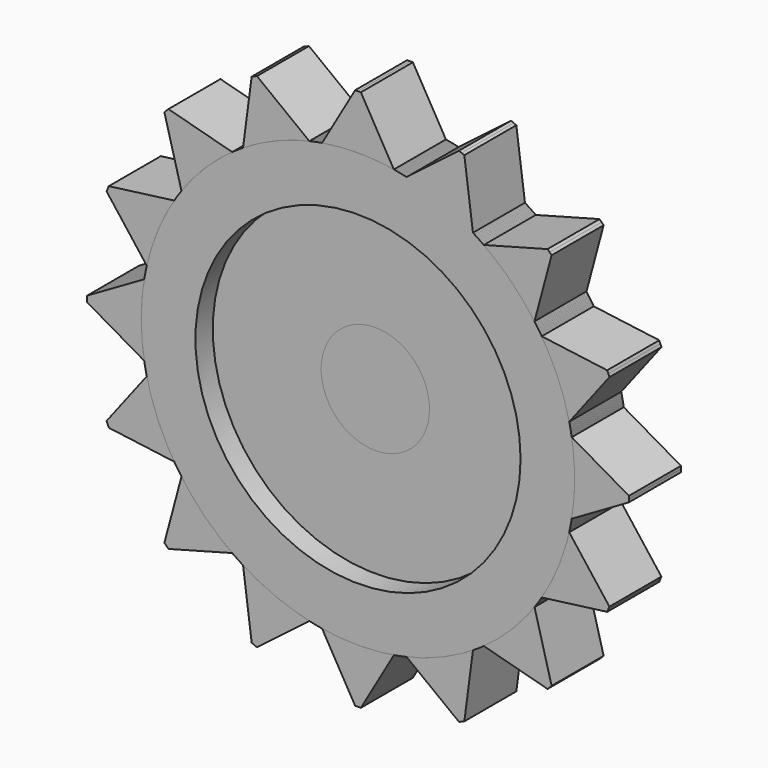
from build123d import *

# Parameters (mm, degrees)
F0_R     = 100
F1_DEPTH = 30
F3_DEPTH = 30
F5_COUNT = 16
F6_R     = 25
F7_DEPTH = 50
F8_R     = 75
F9_DEPTH = 10


# Not quite as in the source:
# - a feature of the source that left no trace in its solid (it failed there, or was rolled back) is left out


with BuildPart() as f1:
    # F0 (on Front) → F1 (new body)
    with BuildSketch(Plane.XZ):
        Circle(F0_R)
    extrude(amount=-F1_DEPTH)

    # F2 (on face) → F3 (join)
    with BuildSketch(Plane.XZ):
        Polygon((1.3260585624, 124.9999999801), (1.4569e-06, 125), (-1.32605566, 125), (-16.5566256365, 98.6198669008), (16.5566285461, 98.6198664123), align=None)
    extrude(amount=-F3_DEPTH)


with BuildPart() as f5_1:
    # F5: instance of F1
    add(f1.part.rotate(Axis((0, 2.4381279945, 0), (0, -1, 0)), 1 * 360 / F5_COUNT))


with BuildPart() as f5_2:
    # F5: instance of F1
    add(f1.part.rotate(Axis((0, 2.4381279945, 0), (0, -1, 0)), 2 * 360 / F5_COUNT))


with BuildPart() as f5_3:
    # F5: instance of F1
    add(f1.part.rotate(Axis((0, 2.4381279945, 0), (0, -1, 0)), 3 * 360 / F5_COUNT))


with BuildPart() as f5_4:
    # F5: instance of F1
    add(f1.part.rotate(Axis((0, 2.4381279945, 0), (0, -1, 0)), 4 * 360 / F5_COUNT))


with BuildPart() as f5_5:
    # F5: instance of F1
    add(f1.part.rotate(Axis((0, 2.4381279945, 0), (0, -1, 0)), 5 * 360 / F5_COUNT))


with BuildPart() as f5_6:
    # F5: instance of F1
    add(f1.part.rotate(Axis((0, 2.4381279945, 0), (0, -1, 0)), 6 * 360 / F5_COUNT))


with BuildPart() as f5_7:
    # F5: instance of F1
    add(f1.part.rotate(Axis((0, 2.4381279945, 0), (0, -1, 0)), 7 * 360 / F5_COUNT))


with BuildPart() as f5_8:
    # F5: instance of F1
    add(f1.part.rotate(Axis((0, 2.4381279945, 0), (0, -1, 0)), 8 * 360 / F5_COUNT))


with BuildPart() as f5_9:
    # F5: instance of F1
    add(f1.part.rotate(Axis((0, 2.4381279945, 0), (0, -1, 0)), 9 * 360 / F5_COUNT))


with BuildPart() as f5_10:
    # F5: instance of F1
    add(f1.part.rotate(Axis((0, 2.4381279945, 0), (0, -1, 0)), 10 * 360 / F5_COUNT))


with BuildPart() as f5_11:
    # F5: instance of F1
    add(f1.part.rotate(Axis((0, 2.4381279945, 0), (0, -1, 0)), 11 * 360 / F5_COUNT))


with BuildPart() as f5_12:
    # F5: instance of F1
    add(f1.part.rotate(Axis((0, 2.4381279945, 0), (0, -1, 0)), 12 * 360 / F5_COUNT))


with BuildPart() as f5_13:
    # F5: instance of F1
    add(f1.part.rotate(Axis((0, 2.4381279945, 0), (0, -1, 0)), 13 * 360 / F5_COUNT))


with BuildPart() as f5_14:
    # F5: instance of F1
    add(f1.part.rotate(Axis((0, 2.4381279945, 0), (0, -1, 0)), 14 * 360 / F5_COUNT))


with BuildPart() as f5_15:
    # F5: instance of F1
    add(f1.part.rotate(Axis((0, 2.4381279945, 0), (0, -1, 0)), 15 * 360 / F5_COUNT))


with BuildPart() as f7:
    # F6 (on face) → F7 (new body)
    with BuildSketch(Plane.XZ):
        Circle(F6_R)
    extrude(amount=-F7_DEPTH)


with BuildPart() as f9_tool:
    # F8 (on face) → F9 (new body)
    with BuildSketch(Plane.XZ):
        Circle(F8_R)
    extrude(amount=-F9_DEPTH)


with BuildPart() as f1_1:
    add(f1.part)

    # F9: cut by f9_tool
    add(f9_tool.part, mode=Mode.SUBTRACT)


with BuildPart() as f5_1_1:
    add(f5_1.part)

    # F9: cut by f9_tool
    add(f9_tool.part, mode=Mode.SUBTRACT)


with BuildPart() as f5_2_1:
    add(f5_2.part)

    # F9: cut by f9_tool
    add(f9_tool.part, mode=Mode.SUBTRACT)


with BuildPart() as f5_3_1:
    add(f5_3.part)

    # F9: cut by f9_tool
    add(f9_tool.part, mode=Mode.SUBTRACT)


with BuildPart() as f5_4_1:
    add(f5_4.part)

    # F9: cut by f9_tool
    add(f9_tool.part, mode=Mode.SUBTRACT)


with BuildPart() as f5_5_1:
    add(f5_5.part)

    # F9: cut by f9_tool
    add(f9_tool.part, mode=Mode.SUBTRACT)


with BuildPart() as f5_6_1:
    add(f5_6.part)

    # F9: cut by f9_tool
    add(f9_tool.part, mode=Mode.SUBTRACT)


with BuildPart() as f5_7_1:
    add(f5_7.part)

    # F9: cut by f9_tool
    add(f9_tool.part, mode=Mode.SUBTRACT)


with BuildPart() as f5_8_1:
    add(f5_8.part)

    # F9: cut by f9_tool
    add(f9_tool.part, mode=Mode.SUBTRACT)


with BuildPart() as f5_9_1:
    add(f5_9.part)

    # F9: cut by f9_tool
    add(f9_tool.part, mode=Mode.SUBTRACT)


with BuildPart() as f5_10_1:
    add(f5_10.part)

    # F9: cut by f9_tool
    add(f9_tool.part, mode=Mode.SUBTRACT)


with BuildPart() as f5_11_1:
    add(f5_11.part)

    # F9: cut by f9_tool
    add(f9_tool.part, mode=Mode.SUBTRACT)


with BuildPart() as f5_12_1:
    add(f5_12.part)

    # F9: cut by f9_tool
    add(f9_tool.part, mode=Mode.SUBTRACT)


with BuildPart() as f5_13_1:
    add(f5_13.part)

    # F9: cut by f9_tool
    add(f9_tool.part, mode=Mode.SUBTRACT)


with BuildPart() as f5_14_1:
    add(f5_14.part)

    # F9: cut by f9_tool
    add(f9_tool.part, mode=Mode.SUBTRACT)


with BuildPart() as f5_15_1:
    add(f5_15.part)

    # F9: cut by f9_tool
    add(f9_tool.part, mode=Mode.SUBTRACT)


with BuildPart() as f7_1:
    add(f7.part)

    # F9: cut by f9_tool
    add(f9_tool.part, mode=Mode.SUBTRACT)


solid = Compound([f1_1.part, f5_1_1.part, f5_2_1.part, f5_3_1.part, f5_4_1.part, f5_5_1.part, f5_6_1.part, f5_7_1.part, f5_8_1.part, f5_9_1.part, f5_10_1.part, f5_11_1.part, f5_12_1.part, f5_13_1.part, f5_14_1.part, f5_15_1.part, f7_1.part])
